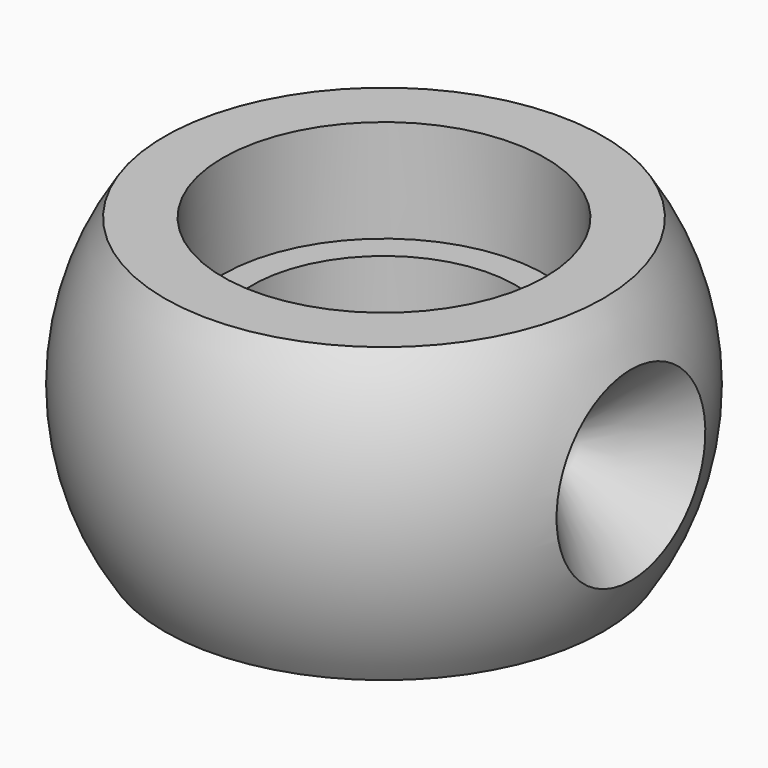
from build123d import *

# Parameters (mm, degrees)
F0_W     = 14.9666295471
F0_H     = 20
F4_R     = 11
F5_DEPTH = 20.001
F6_R     = 12
F6_R_2   = 9
F7_DEPTH = 3


# Not quite as in the source:
# - a pattern or mirror of a feature is missing from the dataset's text; its kind, count and spacing are read off the source's solid


with BuildPart() as f1:
    # F0 (on Front) → F1 (revolve)
    with BuildSketch(Plane.XZ):
        with Locations((7.4833147735, 0)):
            Rectangle(F0_W, F0_H)
        with BuildLine():
            ThreePointArc((14.9666295471, -10), (18, 0), (14.9666295471, 10))
            Line((14.9666295471, 10), (14.9666295471, -10))
        make_face()
    revolve(axis=Axis((0, 0, 0), (0, 0, -1)))

    # F2 (on Top) → F3 (revolve, cut)
    with BuildSketch(Plane.XY):
        Polygon((39.5, 9), (30.5, 0), (39.5, 0), align=None)
    revolve(axis=Axis((35, 0, 0), (-1, 0, 0)), mode=Mode.SUBTRACT)

    # F4 (on face) → F5 (cut, through all)
    with BuildSketch(Plane.XY.offset(10)):
        Circle(F4_R)
    extrude(amount=-F5_DEPTH, mode=Mode.SUBTRACT)

    # F6 (on Top) → F7 (join, symmetric)
    with BuildSketch(Plane.XY):
        Circle(F6_R)
        Circle(F6_R_2, mode=Mode.SUBTRACT)
    extrude(amount=F7_DEPTH, both=True)

    # F8 (on Front) → F9 (revolve, cut)
    with BuildSketch(Plane.XZ):
        Polygon((19.5, 9), (10.5, 0), (19.5, 0), align=None)
    f9 = revolve(axis=Axis((15, 0, 0), (-1, 0, 0)), mode=Mode.SUBTRACT)

    # F9_copies: F9 across plane
    add(f9.mirror(Plane(origin=(0, 0, 0), x_dir=(0, 0, -1), z_dir=(-1, 0, 0))), mode=Mode.SUBTRACT)


solid = f1.part
